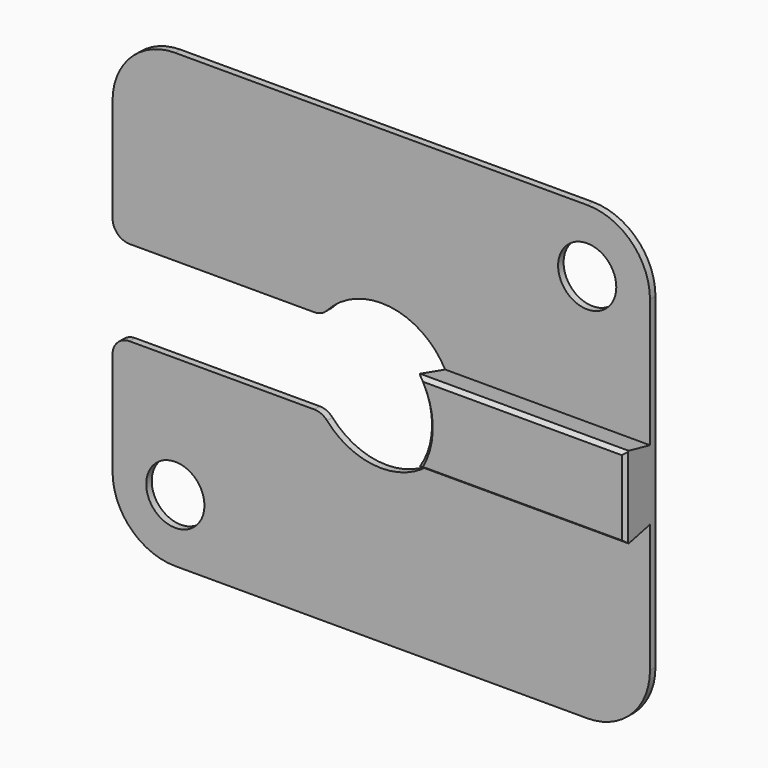
from build123d import *

# Parameters (mm, degrees)
F0_W         = 31.4
F0_H         = 26.4
F0_R         = 1.7
F1_DEPTH     = 0.4
F2_R         = 3.66
F4_DEPTH     = 25
F5_R         = 1
F7_DEPTH     = 2.2
F9_DEPTH     = 25
F10_T1_DEPTH = 13.4922434022
F10_T3_DEPTH = 5.9086731952
F10_T6_ANGLE = 83.9470182362


# Not quite as in the source:
# - a fillet or chamfer that OpenCascade refuses, or shapes differently, is made with other operations: its cross-section is extruded or revolved along the edge and cut away or added


with BuildPart() as f1:
    # F0 (on Front) → F1 (new body)
    with BuildSketch(Plane.XZ):
        Rectangle(F0_W, F0_H)
        with Locations((-12.0318713589, -9.5318713589)):
            Circle(F0_R, mode=Mode.SUBTRACT)
        with Locations((12.0318713589, 9.5318713589)):
            Circle(F0_R, mode=Mode.SUBTRACT)
    extrude(amount=F1_DEPTH)

    # F2
    f2_edges = [f1.edges().sort_by_distance(p)[0] for p in [
        (15.7, -0.2, -13.2),
        (15.7, -0.2, 13.2),
        (-15.7, -0.2, -13.2),
        (-15.7, -0.2, 13.2),
    ]]
    fillet(f2_edges, radius=F2_R)

    # F3 (on Front) → F4 (cut)
    with BuildSketch(Plane.XZ):
        with BuildLine():
            Line((-21.9406711915, -2.5), (-3.4369317712, -2.5))
            ThreePointArc((-3.4369317712, -2.5), (4.25, 0), (-3.4369317712, 2.5))
            Line((-3.4369317712, 2.5), (-21.9406711915, 2.5))
            Line((-21.9406711915, 2.5), (-21.9406711915, -2.5))
        make_face()
    extrude(amount=F4_DEPTH, mode=Mode.SUBTRACT)

    # F5
    f5_edges = [f1.edges().sort_by_distance(p)[0] for p in [
        (-3.436932, -0.2, -2.5),
        (-3.436932, -0.2, 2.5),
        (-15.7, -0.2, 2.5),
        (-15.7, -0.2, -2.5),
    ]]
    fillet(f5_edges, radius=F5_R)

    # F6 (on face) → F7 (join)
    with BuildSketch(Plane(origin=(0, 0, 0), x_dir=(-1, 0, 0), z_dir=(0, 1, 0))):
        with BuildLine():
            Line((-3.4797844761, 2.44), (-15.7, 2.44))
            Line((-15.7, 2.44), (-15.7, -2.44))
            Line((-15.7, -2.44), (-3.4797844761, -2.44))
            ThreePointArc((-3.4797844761, -2.44), (-4.25, 0), (-3.4797844761, 2.44))
        make_face()
    extrude(amount=-F7_DEPTH)

    # F8 (on face) → F9 (cut)
    with BuildSketch(Plane.YZ.offset(15.7)):
        Polygon((-0.4, 2.44), (-2.2, 2.44), (-0.4, 2.04), align=None)
        Polygon((-0.4, -2.04), (-2.2, -2.44), (-0.4, -2.44), align=None)
    extrude(amount=-F9_DEPTH, mode=Mode.SUBTRACT)

    # F10: chamfer of 0.2 on 4 edges, made by hand

    # F10_s2 → F10_t1 (cut)
    with BuildSketch(Plane.YZ.offset(2.8437705369)):
        Polygon((-1.9566139084, 2.3859142019), (-2.2, 2.1906767898), (-2.2, 2.44), align=None)
        Polygon((-2.2, -2.1906767898), (-1.9566139084, -2.3859142019), (-2.2, -2.44), align=None)
    extrude(amount=F10_T1_DEPTH, mode=Mode.SUBTRACT)

    # F10_s4 → F10_t3 (cut)
    with BuildSketch(Plane.XY.offset(-2.9543365976)):
        Polygon((15.5, -2.2), (15.7, -2), (15.7, -2.2), align=None)
    extrude(amount=F10_T3_DEPTH, mode=Mode.SUBTRACT)

    # F10_s5 → F10_t6 (revolve, cut)
    with BuildSketch(Plane(origin=(0, 0, 0), x_dir=(0, 1, 0), z_dir=(-0.6687869395, 0, -0.7434541207))):
        Polygon((-2.2, 4.45), (-2, 4.25), (-2.2, 4.25), align=None)
    revolve(axis=Axis((0, -2.2, 0), (0, -1, 0)), revolution_arc=F10_T6_ANGLE, mode=Mode.SUBTRACT)


solid = f1.part
